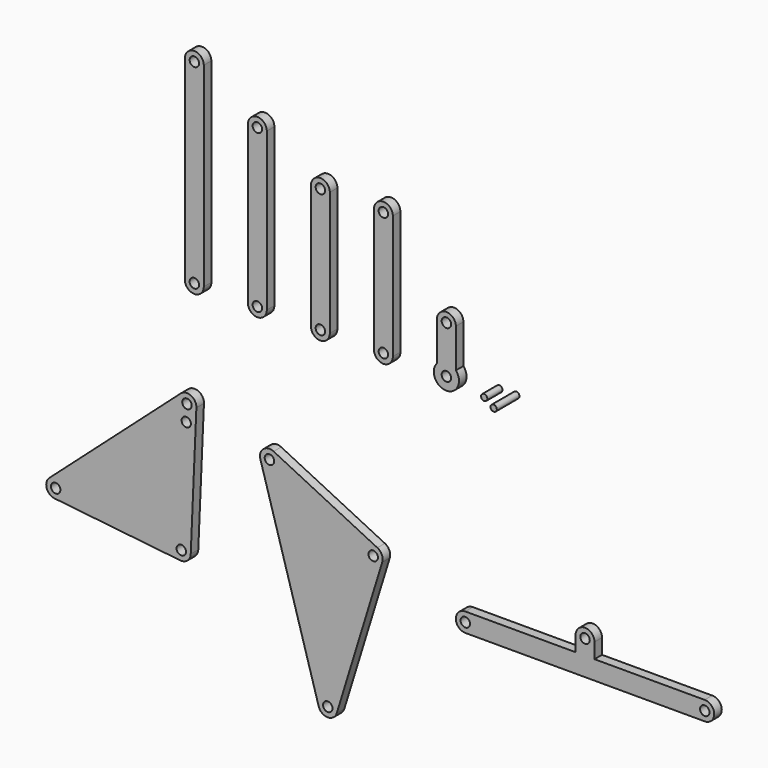
from build123d import *

# Parameters (mm, degrees)
F0_R     = 1.5
F0_R_2   = 1.4708207519
F2_DEPTH = 3
F3_R     = 1
F4_DEPTH = 6
F5_DEPTH = 9


# Not quite as in the source:
# - a feature names something its author has since deleted; it is built from what else it names


with BuildPart() as f2:
    # F0 (on Front) → F2 (new body)
    with BuildSketch(Plane.XZ):
        with BuildLine():
            Line((-91.1504995372, -76.0460597605), (-89.3546715619, -34.5849333663))
            ThreePointArc((-89.3546715619, -34.5849333663), (-91.065599762, -31.7448504778), (-94.3476745872, -32.2153087241))
            Line((-94.3476745872, -32.2153087241), (-136.0080615822, -69.3374336016))
            ThreePointArc((-136.0080615822, -69.3374336016), (-136.8695052558, -72.4916152918), (-134.3368619965, -74.5596253156))
            Line((-134.3368619965, -74.5596253156), (-94.4723029768, -78.8986268323))
            ThreePointArc((-94.4723029768, -78.8986268323), (-92.1932199759, -78.1922130327), (-91.1504995372, -76.0460597605))
        make_face()
        with Locations((-134.0122484167, -71.577239354)):
            Circle(F0_R, mode=Mode.SUBTRACT)
        with Locations((-94.147689397, -75.9162408708)):
            Circle(F0_R, mode=Mode.SUBTRACT)
        with Locations((-92.5760663301, -39.6314388091)):
            Circle(F0_R_2, mode=Mode.SUBTRACT)
        with Locations((-92.3518614217, -34.4551144765)):
            Circle(F0_R, mode=Mode.SUBTRACT)
    extrude(amount=F2_DEPTH)


with BuildPart() as f2b:
    # F0 (on Front) → F2, piece 2 (new body)
    with BuildSketch(Plane.XZ):
        with BuildLine():
            Line((-31.9146860603, -55.0153067294), (-64.8408496002, -38.805502457))
            ThreePointArc((-64.8408496002, -38.805502457), (-68.0972436742, -39.2013842101), (-69.0444341645, -42.342029829))
            Line((-69.0444341645, -42.342029829), (-50.538597649, -105.3818903528))
            ThreePointArc((-50.538597649, -105.3818903528), (-47.6798336145, -107.5368098544), (-44.7929189039, -105.4197521515))
            Line((-44.7929189039, -105.4197521515), (-30.3725918796, -58.5896959001))
            ThreePointArc((-30.3725918796, -58.5896959001), (-30.4851608289, -56.5184149265), (-31.9146860603, -55.0153067294))
        make_face()
        with Locations((-47.660065205, -104.5368749868)):
            Circle(F0_R, mode=Mode.SUBTRACT)
        with Locations((-33.2397381807, -57.7068187353)):
            Circle(F0_R, mode=Mode.SUBTRACT)
        with Locations((-66.1659017205, -41.4970144629)):
            Circle(F0_R, mode=Mode.SUBTRACT)
    extrude(amount=F2_DEPTH)


with BuildPart() as f2c:
    # F0 (on Front) → F2, piece 3 (new body)
    with BuildSketch(Plane.XZ):
        with BuildLine():
            Line((-93, 61.9), (-93, 0))
            ThreePointArc((-93, 0), (-90, -3), (-87, 0))
            Line((-87, 0), (-87, 61.9))
            ThreePointArc((-87, 61.9), (-90, 64.9), (-93, 61.9))
        make_face()
        with Locations((-90, 0)):
            Circle(F0_R, mode=Mode.SUBTRACT)
        with Locations((-90, 61.9)):
            Circle(F0_R, mode=Mode.SUBTRACT)
    extrude(amount=F2_DEPTH)


with BuildPart() as f2d:
    # F0 (on Front) → F2, piece 4 (new body)
    with BuildSketch(Plane.XZ):
        with BuildLine():
            Line((-73, 50), (-73, 0))
            ThreePointArc((-73, 0), (-70, -3), (-67, 0))
            Line((-67, 0), (-67, 50))
            ThreePointArc((-67, 50), (-70, 53), (-73, 50))
        make_face()
        with Locations((-70, 0)):
            Circle(F0_R, mode=Mode.SUBTRACT)
        with Locations((-70, 50)):
            Circle(F0_R, mode=Mode.SUBTRACT)
    extrude(amount=F2_DEPTH)


with BuildPart() as f2e:
    # F0 (on Front) → F2, piece 5 (new body)
    with BuildSketch(Plane.XZ):
        with BuildLine():
            Line((-53, 39.4), (-53, 0))
            ThreePointArc((-53, 0), (-50, -3), (-47, 0))
            Line((-47, 0), (-47, 39.4))
            ThreePointArc((-47, 39.4), (-50, 42.4), (-53, 39.4))
        make_face()
        with Locations((-50, 0)):
            Circle(F0_R, mode=Mode.SUBTRACT)
        with Locations((-50, 39.4)):
            Circle(F0_R, mode=Mode.SUBTRACT)
    extrude(amount=F2_DEPTH)


with BuildPart() as f2f:
    # F0 (on Front) → F2, piece 6 (new body)
    with BuildSketch(Plane.XZ):
        with BuildLine():
            Line((-33, 39.3), (-33, 0))
            ThreePointArc((-33, 0), (-30, -3), (-27, 0))
            Line((-27, 0), (-27, 39.3))
            ThreePointArc((-27, 39.3), (-30, 42.3), (-33, 39.3))
        make_face()
        with Locations((-30, 0)):
            Circle(F0_R, mode=Mode.SUBTRACT)
        with Locations((-30, 39.3)):
            Circle(F0_R, mode=Mode.SUBTRACT)
    extrude(amount=F2_DEPTH)


with BuildPart() as f2g:
    # F0 (on Front) → F2, piece 7 (new body)
    with BuildSketch(Plane.XZ):
        with BuildLine():
            Line((31.0058163851, -63.7388439178), (-3.9941836149, -63.7388439178))
            ThreePointArc((-3.9941836149, -63.7388439178), (-6.9941836149, -66.7388439178), (-3.9941836149, -69.7388439178))
            Line((-3.9941836149, -69.7388439178), (72.0058163851, -69.7388439178))
            ThreePointArc((72.0058163851, -69.7388439178), (75.0055972977, -66.7025882054), (71.9333102557, -63.7397202356))
            Line((71.9333102557, -63.7397202356), (37.0058163851, -63.7397202356))
            Line((37.0058163851, -63.7397202356), (37.0058163851, -58.9388439178))
            ThreePointArc((37.0058163851, -58.9388439178), (34.0058163851, -55.9388439178), (31.0058163851, -58.9388439178))
            Line((31.0058163851, -58.9388439178), (31.0058163851, -63.7388439178))
        make_face()
        with Locations((-3.9941836149, -66.7388439178)):
            Circle(F0_R, mode=Mode.SUBTRACT)
        with Locations((72.0058163851, -66.7388439178)):
            Circle(F0_R, mode=Mode.SUBTRACT)
        with Locations((34.0058163851, -58.9388439178)):
            Circle(F0_R, mode=Mode.SUBTRACT)
    extrude(amount=F2_DEPTH)


with BuildPart() as f2h:
    # F0 (on Front) → F2, piece 8 (new body)
    with BuildSketch(Plane.XZ):
        with BuildLine():
            Line((-7, 2.6457513111), (-7, 15))
            ThreePointArc((-7, 15), (-10, 18), (-13, 15))
            Line((-13, 15), (-13, 2.6457513111))
            ThreePointArc((-13, 2.6457513111), (-10, -4), (-7, 2.6457513111))
        make_face()
        with Locations((-10, 0)):
            Circle(F0_R, mode=Mode.SUBTRACT)
        with Locations((-10, 15)):
            Circle(F0_R, mode=Mode.SUBTRACT)
    extrude(amount=F2_DEPTH)


with BuildPart() as f4:
    # F3 (on Front) → F4 (new body)
    with BuildSketch(Plane.XZ):
        with Locations((4.3974108437, 0)):
            Circle(F3_R)
    extrude(amount=F4_DEPTH)


with BuildPart() as f5:
    # F3 (on Front) → F5 (new body)
    with BuildSketch(Plane.XZ):
        with Locations((9.7946263296, 0)):
            Circle(F3_R)
    extrude(amount=F5_DEPTH)


solid = Compound([f2.part, f2b.part, f2c.part, f2d.part, f2e.part, f2f.part, f2g.part, f2h.part, f4.part, f5.part])
